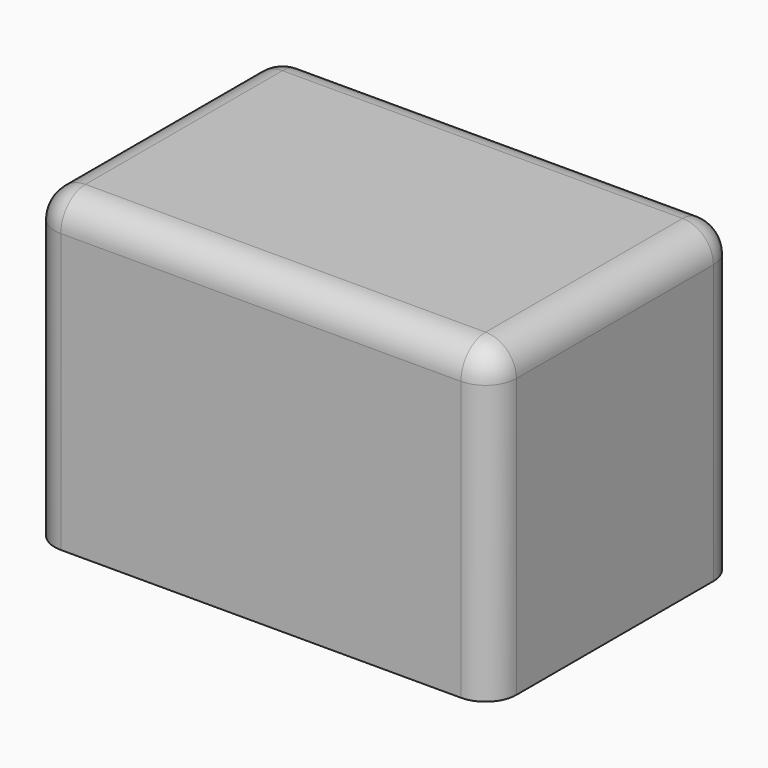
from build123d import *

# Parameters (mm, degrees)
F0_W         = 76.2
F0_H         = 50.8
F1_DEPTH     = 51.054
F2_R         = 5.08
F3_T1_DEPTH  = 58.674
F3_S5_W      = 5.08
F3_S5_H      = 5.08
F3_T6_DEPTH  = 5.08
F3_S11_W     = 5.08
F3_S11_H     = 5.08
F3_T12_DEPTH = 5.08
F3_S17_W     = 5.08
F3_S17_H     = 5.08
F3_T18_DEPTH = 5.08
F3_S23_W     = 5.08
F3_S23_H     = 5.08
F3_T24_DEPTH = 5.08


# Not quite as in the source:
# - a fillet or chamfer that OpenCascade refuses, or shapes differently, is made with other operations: its cross-section is extruded or revolved along the edge and cut away or added


with BuildPart() as f1:
    # F0 (on Top) → F1 (new body)
    with BuildSketch(Plane.XY):
        with Locations((-7.1537382901, -0.4322529342)):
            Rectangle(F0_W, F0_H)
    extrude(amount=F1_DEPTH)

    # F2
    f2_edges = [f1.edges().sort_by_distance(p)[0] for p in [
        (-7.153738, 24.967747, 51.054),
        (-45.253738, -0.432253, 51.054),
        (-7.153738, -25.832253, 51.054),
        (30.946262, -0.432253, 51.054),
    ]]
    fillet(f2_edges, radius=F2_R)

    # F3: fillet of radius 5.08 on 4 edges, made by hand

    # F3_s2 → F3_t1 (cut)
    with BuildSketch(Plane.XY.offset(-12.7)):
        with BuildLine():
            ThreePointArc((-40.1737382901, 24.9677470658), (-43.7658407385, 23.4798495143), (-45.2537382901, 19.8877470658))
            Line((-45.2537382901, 19.8877470658), (-45.2537382901, 24.9677470658))
            Line((-45.2537382901, 24.9677470658), (-40.1737382901, 24.9677470658))
        make_face()
        with BuildLine():
            ThreePointArc((-45.2537382901, -20.7522529342), (-43.7658407385, -24.3443553826), (-40.1737382901, -25.8322529342))
            Line((-40.1737382901, -25.8322529342), (-45.2537382901, -25.8322529342))
            Line((-45.2537382901, -25.8322529342), (-45.2537382901, -20.7522529342))
        make_face()
        with BuildLine():
            ThreePointArc((30.9462617099, -20.7522529342), (29.4583641584, -24.3443553826), (25.8662617099, -25.8322529342))
            Line((25.8662617099, -25.8322529342), (30.9462617099, -25.8322529342))
            Line((30.9462617099, -25.8322529342), (30.9462617099, -20.7522529342))
        make_face()
        with BuildLine():
            ThreePointArc((25.8662617099, 24.9677470658), (29.4583641584, 23.4798495143), (30.9462617099, 19.8877470658))
            Line((30.9462617099, 19.8877470658), (30.9462617099, 24.9677470658))
            Line((30.9462617099, 24.9677470658), (25.8662617099, 24.9677470658))
        make_face()
    extrude(amount=F3_T1_DEPTH, mode=Mode.SUBTRACT)


with BuildPart() as f3_tool4:
    # F3_s5 → F3_t6 (new body)
    with BuildSketch(Plane.XZ.offset(-19.8877470658)):
        with Locations((28.4062617099, 48.514)):
            Rectangle(F3_S5_W, F3_S5_H)
    extrude(amount=-F3_T6_DEPTH)

    # F3_s7 → F3_t8 (revolve, cut)
    with BuildSketch(Plane(origin=(25.8662617099, 19.8877470658, 45.974), x_dir=(-0.7071067812, 0, -0.7071067812), z_dir=(0.7071067812, 0, -0.7071067812))):
        with BuildLine():
            ThreePointArc((0, -5.08), (5.08, 0), (0, 5.08))
            Line((0, 5.08), (0, -5.08))
        make_face()
    revolve(axis=Axis((25.8662617099, 19.8877470658, 45.974), (0, 1, 0)), mode=Mode.SUBTRACT)


with BuildPart() as f1_1:
    add(f1.part)

    # F3_t3: cut F3_tool4
    add(f3_tool4.part, mode=Mode.SUBTRACT)


with BuildPart() as f3_tool10:
    # F3_s11 → F3_t12 (new body)
    with BuildSketch(Plane.YZ.offset(25.8662617099)):
        with Locations((-23.2922529342, 48.514)):
            Rectangle(F3_S11_W, F3_S11_H)
    extrude(amount=F3_T12_DEPTH)

    # F3_s13 → F3_t14 (revolve, cut)
    with BuildSketch(Plane(origin=(25.8662617099, -20.7522529342, 45.974), x_dir=(0, 0.7071067812, -0.7071067812), z_dir=(0, -0.7071067812, -0.7071067812))):
        with BuildLine():
            ThreePointArc((0, -5.08), (5.08, 0), (0, 5.08))
            Line((0, 5.08), (0, -5.08))
        make_face()
    revolve(axis=Axis((25.8662617099, -20.7522529342, 45.974), (1, 0, 0)), mode=Mode.SUBTRACT)


with BuildPart() as f1_2:
    add(f1_1.part)

    # F3_t9: cut F3_tool10
    add(f3_tool10.part, mode=Mode.SUBTRACT)


with BuildPart() as f3_tool16:
    # F3_s17 → F3_t18 (new body)
    with BuildSketch(Plane.YZ.offset(-40.1737382901)):
        with Locations((-23.2922529342, 48.514)):
            Rectangle(F3_S17_W, F3_S17_H)
    extrude(amount=-F3_T18_DEPTH)

    # F3_s19 → F3_t20 (revolve, cut)
    with BuildSketch(Plane(origin=(-40.1737382901, -20.7522529342, 45.974), x_dir=(0, 0.7071067812, -0.7071067812), z_dir=(0, 0.7071067812, 0.7071067812))):
        with BuildLine():
            ThreePointArc((0, -5.08), (5.08, 0), (0, 5.08))
            Line((0, 5.08), (0, -5.08))
        make_face()
    revolve(axis=Axis((-40.1737382901, -20.7522529342, 45.974), (-1, 0, 0)), mode=Mode.SUBTRACT)


with BuildPart() as f1_3:
    add(f1_2.part)

    # F3_t15: cut F3_tool16
    add(f3_tool16.part, mode=Mode.SUBTRACT)


with BuildPart() as f3_tool22:
    # F3_s23 → F3_t24 (new body)
    with BuildSketch(Plane.XZ.offset(-19.8877470658)):
        with Locations((-42.7137382901, 48.514)):
            Rectangle(F3_S23_W, F3_S23_H)
    extrude(amount=-F3_T24_DEPTH)

    # F3_s25 → F3_t26 (revolve, cut)
    with BuildSketch(Plane(origin=(-40.1737382901, 19.8877470658, 45.974), x_dir=(0.7071067812, 0, -0.7071067812), z_dir=(0.7071067812, 0, 0.7071067812))):
        with BuildLine():
            ThreePointArc((0, -5.08), (5.08, 0), (0, 5.08))
            Line((0, 5.08), (0, -5.08))
        make_face()
    revolve(axis=Axis((-40.1737382901, 19.8877470658, 45.974), (0, 1, 0)), mode=Mode.SUBTRACT)


with BuildPart() as f1_4:
    add(f1_3.part)

    # F3_t21: cut F3_tool22
    add(f3_tool22.part, mode=Mode.SUBTRACT)


solid = f1_4.part
